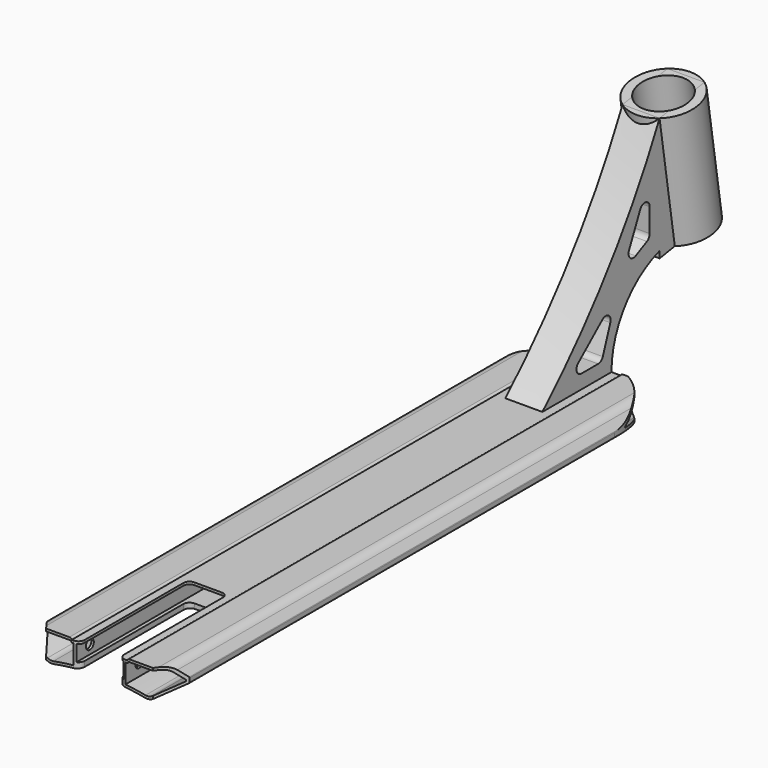
from build123d import *

# Parameters (mm, degrees)
F1_DEPTH       = 250
F2_W           = 38
F2_H           = 13
F3_DEPTH       = 250
F4_T1_DEPTH    = 509.3674969976
F5_R           = 9
F6_R           = 1
F8_DEPTH       = 500.001
F10_DEPTH      = 22.2193051812
F10_DEPTH_BACK = 1.301
F12_DEPTH      = 1.3010001
F12_DEPTH_BACK = 22.219305294
F13_T1_DEPTH   = 2
F13_T6_DEPTH   = 16.7634824315
F13_S7_R       = 200
F13_T8_DEPTH   = 11
F13_T12_DEPTH  = 16.7634824315
F13_S13_R      = 200
F13_T14_DEPTH  = 11
F13_T15_DEPTH  = 27
F13_T17_DEPTH  = 29.2634824315
F15_DEPTH      = 15
F16_R          = 27.5
F17_DEPTH      = 98.7688340595
F19_D          = 40
F21_D          = 8
F21_DEPTH      = 78.5010001
F23_DEPTH      = 72.5010001
F24_R          = 5


# Not quite as in the source:
# - a fillet or chamfer that OpenCascade refuses, or shapes differently, is made with other operations: its cross-section is extruded or revolved along the edge and cut away or added


with BuildPart() as f1:
    # F0 (on Front) → F1 (new body, symmetric)
    with BuildSketch(Plane.XZ):
        with BuildLine():
            Line((22.5, 0), (0, 0))
            Line((0, 0), (-22.5, 0))
            Line((-22.5, 0), (-22.5, 1.3))
            Line((-22.5, 1.3), (-50.0555529561, 1.3))
            Line((-50.0555529561, 1.3), (-57.5, -8.7))
            Line((-57.5, -8.7), (-57.5, -12.7))
            Line((-57.5, -12.7), (-40.1794919243, -22.7))
            ThreePointArc((-40.1794919243, -22.7), (0, -18.6224551416), (40.1794919243, -22.7))
            Line((40.1794919243, -22.7), (57.5, -12.7))
            Line((57.5, -12.7), (57.5, -8.7))
            Line((57.5, -8.7), (50.0555529561, 1.3))
            Line((50.0555529561, 1.3), (22.5, 1.3))
            Line((22.5, 1.3), (22.5, 0))
        make_face()
    extrude(amount=F1_DEPTH, both=True)

    # F2 (on Front) → F3 (cut, symmetric)
    with BuildSketch(Plane.XZ):
        with Locations((0, -8.5)):
            Rectangle(F2_W, F2_H)
    extrude(amount=F3_DEPTH, both=True, mode=Mode.SUBTRACT)

    # F4: fillet of radius 2 on 2 edges, made by hand

    # F4_s2 → F4_t1 (cut)
    with BuildSketch(Plane.XZ.offset(-254.6837484988)):
        with BuildLine():
            ThreePointArc((-24.3734993995, 1.3), (-23.2333239744, 0.9431676725), (-22.5, 0))
            Line((-22.5, 0), (-22.5, 1.3))
            Line((-22.5, 1.3), (-24.3734993995, 1.3))
        make_face()
        with BuildLine():
            ThreePointArc((24.3734993995, 1.3), (23.2333239744, 0.9431676725), (22.5, 0))
            Line((22.5, 0), (22.5, 1.3))
            Line((22.5, 1.3), (24.3734993995, 1.3))
        make_face()
    extrude(amount=F4_T1_DEPTH, mode=Mode.SUBTRACT)

    # F5
    f5_edges = [f1.edges().sort_by_distance(p)[0] for p in [
        (-50.055553, 0, 1.3),
        (-40.179492, 0, -22.7),
        (50.055553, 0, 1.3),
        (40.179492, 0, -22.7),
    ]]
    fillet(f5_edges, radius=F5_R)

    # F6
    f6_edges = [f1.edges().sort_by_distance(p)[0] for p in [
        (57.5, 0, -8.7),
        (57.5, 0, -12.7),
        (-57.5, 0, -8.7),
        (-57.5, 0, -12.7),
    ]]
    fillet(f6_edges, radius=F6_R)

    # F7 (on face) → F8 (cut, through all)
    with BuildSketch(Plane.XZ.offset(250)):
        with BuildLine():
            ThreePointArc((-42.1022690923, -19.2804830077), (-39.7790673433, -20.1186780608), (-37.3093701274, -20.0978700124))
            ThreePointArc((-37.3093701274, -20.0978700124), (-29.1789785809, -18.7410222645), (-21, -17.7170047426))
            Line((-21, -17.7170047426), (-21, -2))
            Line((-21, -2), (-22.5, -2))
            ThreePointArc((-22.5, -2), (-23.2333239744, -1.0568323275), (-24.3734993995, -0.7))
            Line((-24.3734993995, -0.7), (-45.5354825976, -0.7))
            ThreePointArc((-45.5354825976, -0.7), (-48.677132627, -1.4445995258), (-51.1504194786, -3.5199899734))
            Line((-51.1504194786, -3.5199899734), (-55.9653979223, -9.9878692065))
            ThreePointArc((-55.9653979223, -9.9878692065), (-56.1426029011, -10.7872397993), (-55.6632640822, -11.4510388998))
            Line((-55.6632640822, -11.4510388998), (-42.1022690923, -19.2804830077))
        make_face()
        with BuildLine():
            Line((21, -2), (21, -17.7170047426))
            ThreePointArc((21, -17.7170047426), (29.1789785809, -18.7410222645), (37.3093701274, -20.0978700124))
            ThreePointArc((37.3093701274, -20.0978700124), (39.7790673433, -20.1186780608), (42.1022690923, -19.2804830077))
            Line((42.1022690923, -19.2804830077), (55.6632640822, -11.4510388998))
            ThreePointArc((55.6632640822, -11.4510388998), (56.1426029011, -10.7872397993), (55.9653979223, -9.9878692065))
            Line((55.9653979223, -9.9878692065), (51.1504194786, -3.5199899734))
            ThreePointArc((51.1504194786, -3.5199899734), (48.677132627, -1.4445995258), (45.5354825976, -0.7))
            Line((45.5354825976, -0.7), (24.3734993995, -0.7))
            ThreePointArc((24.3734993995, -0.7), (23.2333239744, -1.0568323275), (22.5, -2))
            Line((22.5, -2), (21, -2))
        make_face()
    extrude(amount=-F8_DEPTH, mode=Mode.SUBTRACT)

    # F9 (on Top) → F10 (cut, two sides)
    with BuildSketch(Plane.XY) as f10_sk:
        with BuildLine():
            ThreePointArc((-57.5, 200), (0, 257.5), (57.5, 200))
            Line((57.5, 200), (57.5, 280))
            Line((57.5, 280), (-57.5, 280))
            Line((-57.5, 280), (-57.5, 200))
        make_face()
    extrude(amount=-F10_DEPTH, mode=Mode.SUBTRACT)
    extrude(f10_sk.sketch, amount=F10_DEPTH_BACK, mode=Mode.SUBTRACT)

    # F11 (on Top) → F12 (cut, two sides)
    with BuildSketch(Plane.XY) as f12_sk:
        Polygon((-43.2975540478, -250), (-68, -216), (-68, -346), (68, -346), (68, -216), (43.2975540478, -250), (16, -250), (16, -140), (-16, -140), (-16, -250), align=None)
    extrude(amount=F12_DEPTH, mode=Mode.SUBTRACT)
    extrude(f12_sk.sketch, amount=-F12_DEPTH_BACK, mode=Mode.SUBTRACT)

    # F13: fillet of radius 5 on 8 edges, made by hand

    # F13_s2 → F13_t1 (join)
    with BuildSketch(Plane.XY.offset(-2)):
        with BuildLine():
            ThreePointArc((16, -145), (14.5355339059, -141.4644660941), (11, -140))
            Line((11, -140), (16, -140))
            Line((16, -140), (16, -145))
        make_face()
        with BuildLine():
            ThreePointArc((-11, -140), (-14.5355339059, -141.4644660941), (-16, -145))
            Line((-16, -145), (-16, -140))
            Line((-16, -140), (-11, -140))
        make_face()
    extrude(amount=F13_T1_DEPTH)


with BuildPart() as f13_tool4:
    # F13_s5 → F13_t6 (new body)
    with BuildSketch(Plane.XY.offset(-31.7634824315)):
        with BuildLine():
            ThreePointArc((-16, -145), (-14.5355339059, -141.4644660941), (-11, -140))
            Line((-11, -140), (-16, -140))
            Line((-16, -140), (-16, -145))
        make_face()
    extrude(amount=F13_T6_DEPTH)

    # F13_s7 → F13_t8 (cut, symmetric)
    with BuildSketch(Plane.XZ.offset(142.5)):
        with Locations((0, -218.6224551416)):
            Circle(F13_S7_R)
    extrude(amount=F13_T8_DEPTH, both=True, mode=Mode.SUBTRACT)


with BuildPart() as f1_1:
    add(f1.part)

    # F13_t3: union F13_tool4
    add(f13_tool4.part)


with BuildPart() as f13_tool10:
    # F13_s11 → F13_t12 (new body)
    with BuildSketch(Plane.XY.offset(-31.7634824315)):
        with BuildLine():
            ThreePointArc((16, -145), (14.5355339059, -141.4644660941), (11, -140))
            Line((11, -140), (16, -140))
            Line((16, -140), (16, -145))
        make_face()
    extrude(amount=F13_T12_DEPTH)

    # F13_s13 → F13_t14 (cut, symmetric)
    with BuildSketch(Plane.XZ.offset(142.5)):
        with Locations((0, -218.6224551416)):
            Circle(F13_S13_R)
    extrude(amount=F13_T14_DEPTH, both=True, mode=Mode.SUBTRACT)


with BuildPart() as f1_2:
    add(f1_1.part)

    # F13_t9: union F13_tool10
    add(f13_tool10.part)

    # F13_s16 → F13_t15 (cut)
    with BuildSketch(Plane.XY.offset(-14.5)):
        with BuildLine():
            ThreePointArc((-21, -250), (-17.4644660941, -248.5355339059), (-16, -245))
            Line((-16, -245), (-16, -250))
            Line((-16, -250), (-21, -250))
        make_face()
        with BuildLine():
            ThreePointArc((21, -250), (17.4644660941, -248.5355339059), (16, -245))
            Line((16, -245), (16, -250))
            Line((16, -250), (21, -250))
        make_face()
    extrude(amount=F13_T15_DEPTH, mode=Mode.SUBTRACT)

    # F13_s18 → F13_t17 (cut)
    with BuildSketch(Plane.XY.offset(-31.7634824315)):
        with BuildLine():
            ThreePointArc((-21, -250), (-17.4644660941, -248.5355339059), (-16, -245))
            Line((-16, -245), (-16, -250))
            Line((-16, -250), (-21, -250))
        make_face()
        with BuildLine():
            ThreePointArc((21, -250), (17.4644660941, -248.5355339059), (16, -245))
            Line((16, -245), (16, -250))
            Line((16, -250), (21, -250))
        make_face()
    extrude(amount=F13_T17_DEPTH, mode=Mode.SUBTRACT)

    # F14 (on Right) → F15 (join, symmetric)
    with BuildSketch(Plane.YZ):
        with BuildLine():
            ThreePointArc((298.7642824058, 161.3), (246.7870939845, 75.1977749327), (180, 0))
            Line((180, 0), (250, 0))
            ThreePointArc((250, 0), (263.4911501108, 41.3128295352), (298.7642824058, 66.7011566486))
            Line((298.7642824058, 66.7011566486), (298.7642824058, 61.3))
            Line((298.7642824058, 61.3), (344.1979460732, 68.4959853919))
            Line((344.1979460732, 68.4959853919), (344.1979460732, 168.4959853919))
            Line((344.1979460732, 168.4959853919), (298.7642824058, 161.3))
        make_face()
    extrude(amount=F15_DEPTH, both=True)

    # F16 (on face) → F17 (join, through all)
    with BuildSketch(Plane(origin=(0, -17.6109382026, 111.1910877514), x_dir=(1, 0, 0), z_dir=(0, -0.156434465, 0.9876883406))):
        with Locations((0, 343.3188775295)):
            Circle(F16_R)
    extrude(amount=-F17_DEPTH)

    # F19 (through all)
    with Locations(Plane(origin=(0, -17.6109382026, 111.1910877514), x_dir=(1, 0, 0), z_dir=(0, -0.156434465, 0.9876883406))):
        with Locations((0, 343.3188775294)):
            Hole(F19_D / 2)

    # F21 (through all, one way)
    with BuildSketch(Plane.YZ.offset(21)):
        with Locations((-236, -7.7170047426)):
            Circle(F21_D / 2)
    extrude(amount=-F21_DEPTH, mode=Mode.SUBTRACT)

    # F22 (on face) → F23 (cut, through all)
    with BuildSketch(Plane.YZ.offset(15)):
        Polygon((255.3909064497, 53.5861679354), (206, 11.3), (240, 11.3), align=None)
        Polygon((288.7269891839, 79.9595514464), (288.7269891839, 124.9595514464), (261.8157467862, 66.7011566486), align=None)
    extrude(amount=-F23_DEPTH, mode=Mode.SUBTRACT)

    # F24
    f24_edges = [f1_2.edges().sort_by_distance(p)[0] for p in [
        (0, 288.726989, 79.959551),
        (0, 261.815747, 66.701157),
        (0, 288.726989, 124.959551),
        (0, 255.390906, 53.586168),
        (0, 240, 11.3),
        (0, 206, 11.3),
    ]]
    fillet(f24_edges, radius=F24_R)


solid = f1_2.part
